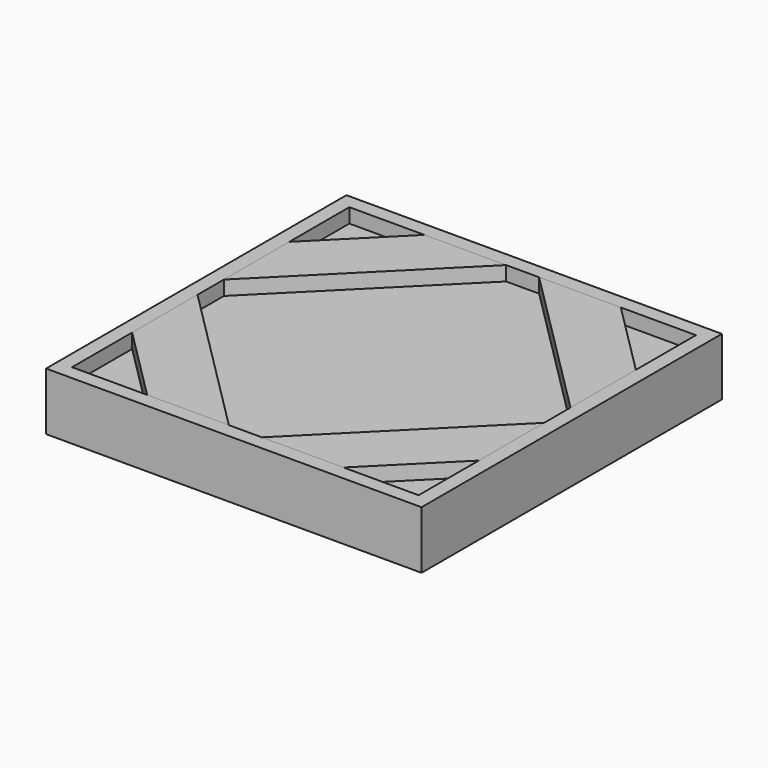
from build123d import *

# Parameters (mm, degrees)
F0_W          = 600
F0_H          = 600
F1_DEPTH      = 15
F3_W          = 650
F3_H          = 650
F3_W_2        = 600
F3_H_2        = 600
F4_DEPTH      = 75
F4_DEPTH_BACK = 25
F6_DEPTH      = 25


with BuildPart() as f1:
    # F0 (on Top) → F1 (new body)
    with BuildSketch(Plane.XY):
        Rectangle(F0_W, F0_H)
    extrude(amount=F1_DEPTH)


with BuildPart() as f4:
    # F3 (on face) → F4 (new body, two sides)
    with BuildSketch(Plane.XY.offset(15)) as f4_sk:
        Rectangle(F3_W, F3_H)
        Rectangle(F3_W_2, F3_H_2, mode=Mode.SUBTRACT)
    extrude(amount=-F4_DEPTH)
    extrude(f4_sk.sketch, amount=F4_DEPTH_BACK)


with BuildPart() as f6:
    # F5 (on face) → F6 (new body)
    with BuildSketch(Plane.XY.offset(40)):
        Polygon((-28.5786437627, 300), (-170, 300), (-300, 170), (-300, 28.5786437627), align=None)
    extrude(amount=-F6_DEPTH)


with BuildPart() as f6b:
    # F5 (on face) → F6, piece 2 (new body)
    with BuildSketch(Plane.XY.offset(40)):
        Polygon((300, 170), (170, 300), (28.5786437627, 300), (300, 28.5786437627), align=None)
    extrude(amount=-F6_DEPTH)


with BuildPart() as f6c:
    # F5 (on face) → F6, piece 3 (new body)
    with BuildSketch(Plane.XY.offset(40)):
        Polygon((170, -300), (300, -170), (300, -28.5786437627), (28.5786437627, -300), align=None)
    extrude(amount=-F6_DEPTH)


with BuildPart() as f6d:
    # F5 (on face) → F6, piece 4 (new body)
    with BuildSketch(Plane.XY.offset(40)):
        Polygon((-28.5786437627, -300), (-300, -28.5786437627), (-300, -170), (-170, -300), align=None)
    extrude(amount=-F6_DEPTH)


solid = Compound([f1.part, f4.part, f6.part, f6b.part, f6c.part, f6d.part])
